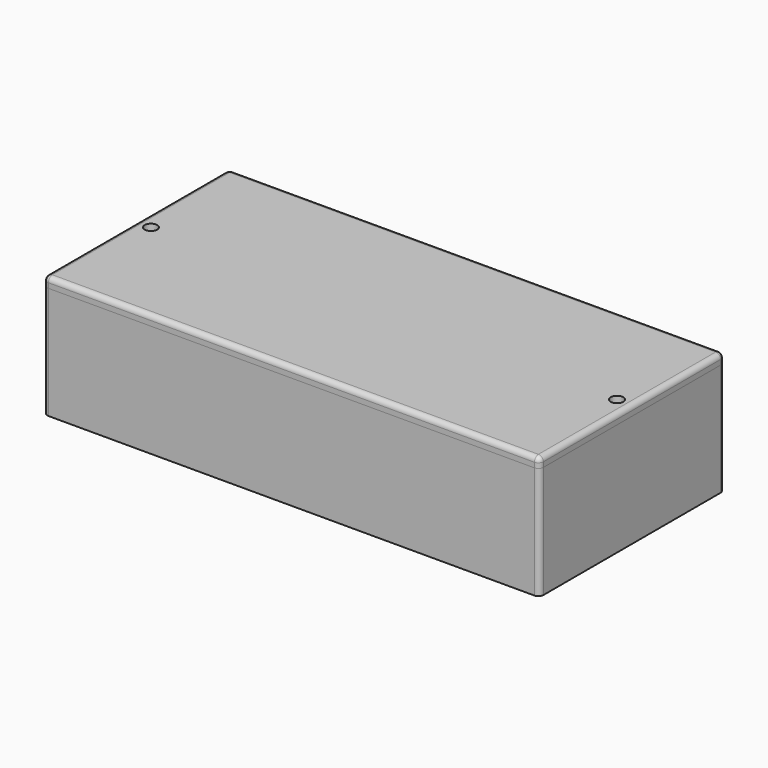
from build123d import *

# Parameters (mm, degrees)
F0_W     = 150
F0_H     = 70
F0_R     = 1.875
F1_DEPTH = 2
F2_R     = 1.25
F3_DEPTH = 32
F4_W     = 150
F4_H     = 70
F4_R     = 1.9
F5_DEPTH = 3
F7_DEPTH = 2
F8_R     = 1.5
F8_2_R   = 1.5
F9_R     = 0.99999


# Not quite as in the source:
# - a fillet or chamfer is up to 0.001 mm smaller than in the source, because OpenCascade refuses the exact size


with BuildPart() as f1:
    # F0 (on Top) → F1 (new body)
    with BuildSketch(Plane.XY):
        Rectangle(F0_W, F0_H)
        with Locations((-67, -27)):
            Circle(F0_R, mode=Mode.SUBTRACT)
        with Locations((67, -27)):
            Circle(F0_R, mode=Mode.SUBTRACT)
        with Locations((-67, 27)):
            Circle(F0_R, mode=Mode.SUBTRACT)
        with Locations((67, 27)):
            Circle(F0_R, mode=Mode.SUBTRACT)
    extrude(amount=-F1_DEPTH)

    # F2 (on Top) → F3 (join)
    with BuildSketch(Plane.XY):
        with BuildLine():
            Line((75, -35), (75, 35))
            Line((75, 35), (-75, 35))
            Line((-75, 35), (-75, 27))
            Line((-75, 27), (-73, 27))
            Line((-73, 27), (-73, 33))
            Line((-73, 33), (73, 33))
            Line((73, 33), (73, 2.4534972628))
            Line((73, 2.4534972628), (70.5469351619, 2.4995593793))
            ThreePointArc((70.5469351619, 2.4995593793), (68.0000628641, 0.0177289705), (70.5114796409, -2.4999736434))
            Line((70.5114796409, -2.4999736434), (73, -2.4999736434))
            Line((73, -2.4999736434), (73, -33))
            Line((73, -33), (-73, -33))
            Line((-73, -33), (-73, -2.4990718681))
            Line((-73, -2.4990718681), (-70.5681160628, -2.4990718681))
            Line((-70.5681160628, -2.4990718681), (-70.4318839372, -2.4990718681))
            ThreePointArc((-70.4318839372, -2.4990718681), (-68.0003076438, -0.0392189257), (-70.3535183815, 2.4957049376))
            Line((-70.3535183815, 2.4957049376), (-70.6464816185, 2.4957049376))
            Line((-70.6464816185, 2.4957049376), (-73, 2.4957049376))
            Line((-73, 2.4957049376), (-73, 22))
            Line((-73, 22), (-75, 22))
            Line((-75, 22), (-75, -35))
            Line((-75, -35), (75, -35))
        make_face()
        with Locations((-70.5, 0)):
            Circle(F2_R, mode=Mode.SUBTRACT)
        with Locations((70.5, 0)):
            Circle(F2_R, mode=Mode.SUBTRACT)
    extrude(amount=F3_DEPTH)

    # F8
    f8_edges = [f1.edges().sort_by_distance(p)[0] for p in [
        (-75, -35, 15),
        (75, -35, 15),
        (75, 35, 15),
        (-75, 35, 15),
    ]]
    fillet(f8_edges, radius=F8_R)

    # F9 (radius 1 in the source; OpenCascade refuses exactly that, so slightly less here)
    f9_edges = [f1.edges().sort_by_distance(p)[0] for p in [
        (-75, 22, 16),
        (-73, 22, 16),
        (-75, 27, 16),
        (-73, 27, 16),
    ]]
    fillet(f9_edges, radius=F9_R)


with BuildPart() as f5:
    # F4 (on face) → F5 (new body)
    with BuildSketch(Plane.XY.offset(32)):
        Rectangle(F4_W, F4_H)
        with Locations((-70.5, 0)):
            Circle(F4_R, mode=Mode.SUBTRACT)
        with Locations((70.5, 0)):
            Circle(F4_R, mode=Mode.SUBTRACT)
    extrude(amount=F5_DEPTH)

    # F6 (on face) → F7 (join)
    with BuildSketch(Plane.XY.offset(32)):
        Polygon((-72, -3), (-72, -32), (72, -32), (72, -2.9580398915), (70, -2.9580398915), (70, -30), (-70, -30), (-70, -3), align=None)
        Polygon((72, 32), (-72, 32), (-72, 2.9580398915), (-70, 2.9580398915), (-70, 30), (70, 30), (70, 2.9580398915), (72, 2.9580398915), align=None)
    extrude(amount=-F7_DEPTH)

    # F8#2
    f8_2_edges = [f5.edges().sort_by_distance(p)[0] for p in [
        (-75, -35, 33.5),
        (-75, 35, 33.5),
        (75, 35, 33.5),
        (75, -35, 33.5),
        (-75, 0, 35),
        (0, 35, 35),
        (75, 0, 35),
        (0, -35, 35),
    ]]
    fillet(f8_2_edges, radius=F8_2_R)


solid = Compound([f1.part, f5.part])
